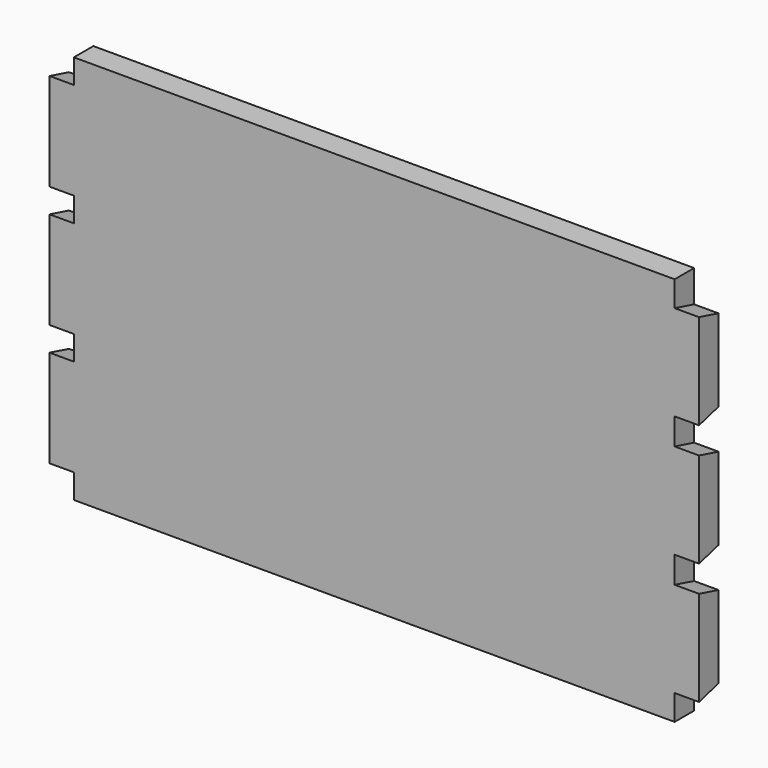
from build123d import *

# Parameters (mm, degrees)
F0_W     = 508
F0_H     = 304.8
F1_DEPTH = 9.525
F3_DEPTH = 19.05
F5_DEPTH = 19.05


# Not quite as in the source:
# - a feature names something its author has since deleted; it is built from what else it names


with BuildPart() as f1:
    # F0 (on Front) → F1 (new body, symmetric)
    with BuildSketch(Plane.XZ):
        Rectangle(F0_W, F0_H)
    extrude(amount=F1_DEPTH, both=True)

    # F2 (on face) → F3 (cut)
    with BuildSketch(Plane(origin=(-254, 0, 0), x_dir=(0, -1, 0), z_dir=(-1, 0, 0))):
        Polygon((-9.525, 128.2455678842), (9.525, 133.35), (9.525, 152.4), (-9.525, 152.4), align=None)
        Polygon((9.525, 38.1), (9.525, 57.15), (-9.525, 62.2544321158), (-9.525, 32.9955678842), align=None)
        Polygon((9.525, -57.15), (9.525, -38.1), (-9.525, -32.9955678842), (-9.525, -62.2544321158), align=None)
        Polygon((9.525, -152.4), (9.525, -133.35), (-9.525, -128.2455678842), (-9.525, -152.4), align=None)
    extrude(amount=-F3_DEPTH, mode=Mode.SUBTRACT)

    # F4 (on face) → F5 (cut)
    with BuildSketch(Plane.YZ.offset(254)):
        Polygon((-9.525, 132.499261314), (9.525, 127.3948291982), (9.525, 152.4), (-9.525, 152.4), align=None)
        Polygon((9.525, 32.1448291982), (9.525, 63.1051708018), (-9.525, 58.000738686), (-9.525, 37.249261314), align=None)
        Polygon((9.525, -63.1051708018), (9.525, -32.1448291982), (-9.525, -37.249261314), (-9.525, -58.000738686), align=None)
        Polygon((9.525, -152.4), (9.525, -127.3948291982), (-9.525, -132.499261314), (-9.525, -152.4), align=None)
    extrude(amount=-F5_DEPTH, mode=Mode.SUBTRACT)


solid = f1.part
